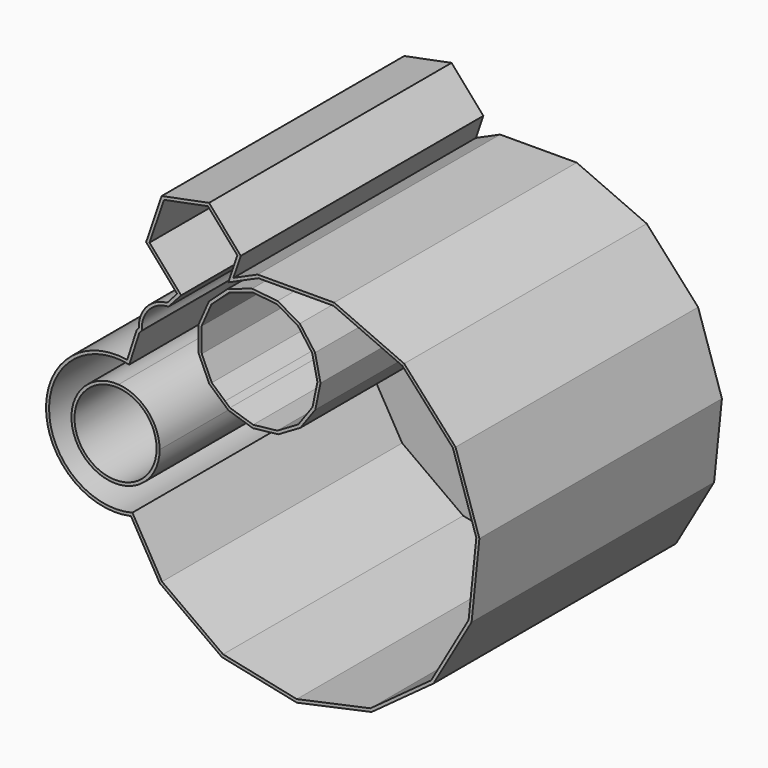
from build123d import *

# Parameters (mm, degrees)
F1_DEPTH = 254
F2_T     = -2.54


with BuildPart() as f1:
    # F0 (on Front) → F1 (new body)
    with BuildSketch(Plane.XZ):
        with BuildLine():
            ThreePointArc((-243.4017726194, -88.5928585449), (-220.6078758628, -99.4306883092), (-211.3480547487, -122.9099556804))
            ThreePointArc((-211.3480547487, -122.9099556804), (-220.0765697788, -145.8071744938), (-241.8322543151, -157.0836896635))
            Line((-241.8322543151, -157.0836896635), (-240.887536248, -165.8666205301))
            Line((-240.887536248, -165.8666205301), (-232.8631227599, -179.6876024772))
            ThreePointArc((-232.8631227599, -179.6876024772), (-200.2497848188, -159.2393547198), (-187.5244002098, -122.9099556804))
            ThreePointArc((-187.5244002098, -122.9099556804), (-201.2534802405, -85.358063124), (-235.9657806801, -65.5164787306))
            Line((-235.9657806801, -65.5164787306), (-243.4017726194, -88.5928585449))
        make_face()
        with BuildLine():
            ThreePointArc((-241.8322543151, -157.0836896635), (-280.1330429902, -123.6979818064), (-243.4017726194, -88.5928585449))
            Line((-243.4017726194, -88.5928585449), (-235.9657806801, -65.5164787306))
            ThreePointArc((-235.9657806801, -65.5164787306), (-303.9442391321, -124.4915476748), (-232.8631227599, -179.6876024772))
            Line((-232.8631227599, -179.6876024772), (-240.887536248, -165.8666205301))
            Line((-240.887536248, -165.8666205301), (-241.8322543151, -157.0836896635))
        make_face()
        with BuildLine():
            Line((-228.0725515097, -41.0211382589), (-235.9657806801, -65.5164787306))
            ThreePointArc((-235.9657806801, -65.5164787306), (-201.2534802405, -85.358063124), (-187.5244002098, -122.9099556804))
            ThreePointArc((-187.5244002098, -122.9099556804), (-200.2497848188, -159.2393547198), (-232.8631227599, -179.6876024772))
            Line((-232.8631227599, -179.6876024772), (-208.6762458399, -221.3462719571))
            Line((-208.6762458399, -221.3462719571), (-156.6841606223, -258.9279433801))
            Line((-156.6841606223, -258.9279433801), (-93.9011844627, -272.1134223913))
            Line((-93.9011844627, -272.1134223913), (-31.1830643044, -258.6228198834))
            Line((-31.1830643044, -258.6228198834), (20.6256671009, -220.7887835882))
            Line((20.6256671009, -220.7887835882), (52.5668094258, -165.1531620926))
            Line((52.5668094258, -165.1531620926), (59.117448986, -101.335859787))
            Line((59.117448986, -101.335859787), (39.144920691, -40.3714680019))
            Line((39.144920691, -40.3714680019), (-3.8973438724, 7.1987160788))
            Line((-3.8973438724, 7.1987160788), (-62.5669461344, 33.1493754661))
            Line((-62.5669461344, 33.1493754661), (-126.7193788673, 32.9934053975))
            Line((-126.7193788673, 32.9934053975), (-147.0301676591, 23.8912264385))
            Line((-147.0301676591, 23.8912264385), (-151.3720759465, 11.1500154879))
            Line((-151.3720759465, 11.1500154879), (-150.3917100203, 12.0439557169))
            Line((-150.3917100203, 12.0439557169), (-131.0449616301, 18.4647337066))
            Line((-131.0449616301, 18.4647337066), (-110.7592618326, 16.461374779))
            Line((-110.7592618326, 16.461374779), (-93.0421924126, 6.3802778925))
            Line((-93.0421924126, 6.3802778925), (-80.9571956273, -10.0354437172))
            Line((-80.9571956273, -10.0354437172), (-76.5938772097, -29.9473626517))
            Line((-76.5938772097, -29.9473626517), (-80.7066945537, -49.9125272331))
            Line((-80.7066945537, -49.9125272331), (-92.5845041767, -66.4787791275))
            Line((-92.5845041767, -66.4787791275), (-110.1735248884, -76.7816628826))
            Line((-110.1735248884, -76.7816628826), (-130.4324552165, -79.0397162985))
            Line((-130.4324552165, -79.0397162985), (-149.8583420607, -72.8625014256))
            Line((-149.8583420607, -72.8625014256), (-153.9562515064, -69.2190774413))
            Line((-153.9562515064, -69.2190774413), (-165.0922731069, -59.3181148339))
            Line((-165.0922731069, -59.3181148339), (-173.5001632814, -40.7485040119))
            Line((-173.5001632814, -40.7485040119), (-173.6282119898, -20.3645233703))
            Line((-173.6282119898, -20.3645233703), (-165.4542784469, -1.6907483448))
            Line((-165.4542784469, -1.6907483448), (-160.8135918091, 2.5408312775))
            Line((-160.8135918091, 2.5408312775), (-193.497810345, -3.9201981196))
            Line((-193.497810345, -3.9201981196), (-194.1558035405, -3.1681041604))
            Line((-194.1558035405, -3.1681041604), (-202.5303474039, -12.5145749574))
            Line((-202.5303474039, -12.5145749574), (-226.2911018969, -39.0329384174))
            Line((-226.2911018969, -39.0329384174), (-228.0725515097, -41.0211382589))
        make_face()
        with BuildLine():
            ThreePointArc((-202.5303474039, -12.5145749574), (-219.6834854839, -21.0493031647), (-226.2911018969, -39.0329384174))
            Line((-226.2911018969, -39.0329384174), (-202.5303474039, -12.5145749574))
        make_face()
        Polygon((-185.2621036451, 6.7577745149), (-194.1558035405, -3.1681041604), (-193.497810345, -3.9201981196), (-160.8135918091, 2.5408312775), (-151.3720759465, 11.1500154879), (-147.0301676591, 23.8912264385), align=None)
        Polygon((-220.1187830788, 26.5078867238), (-194.1558035405, -3.1681041604), (-185.2621036451, 6.7577745149), (-147.0301676591, 23.8912264385), (-140.7948214191, 42.1886792022), (-167.4157941529, 72.6167640457), (-207.0777749827, 64.7763678065), align=None)
    extrude(amount=F1_DEPTH)

    # F2
    f2_openings = [f1.faces().sort_by_distance(p)[0] for p in [
        (-102.007505, -254, -118.633515),
    ]]
    offset(amount=F2_T, openings=f2_openings, kind=Kind.INTERSECTION)


solid = f1.part
